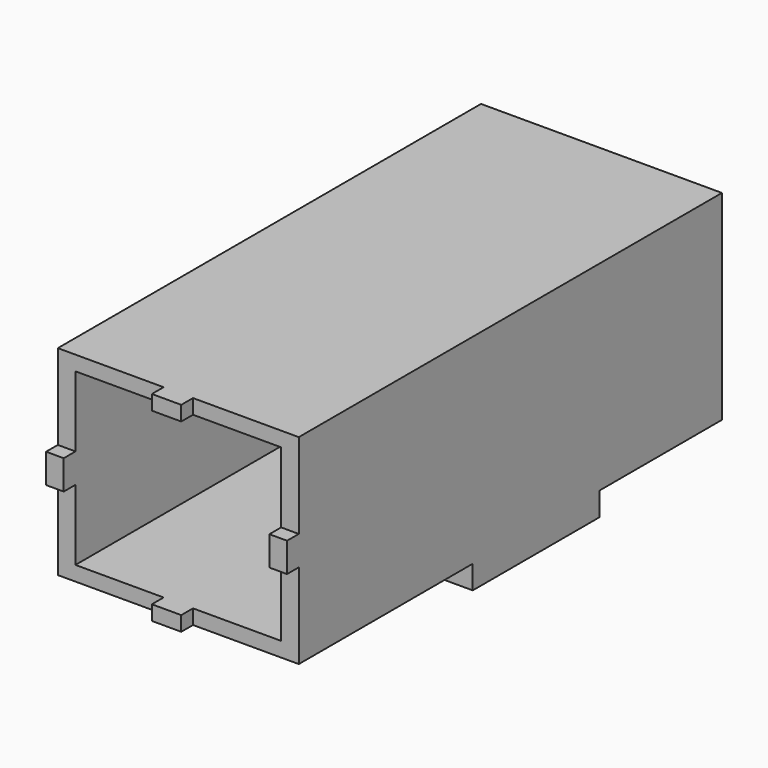
from build123d import *

# Parameters (mm, degrees)
F0_W           = 41
F0_H           = 90
F1_DEPTH       = 34
F2_W           = 35
F2_H           = 29
F3_DEPTH       = 86
F4_W           = 7
F4_H           = 6
F4_R           = 1.55
F4_R_2         = 4
F5_DEPTH       = 4
F6_W           = 5
F6_H           = 2.5
F6_W_2         = 3
F6_H_2         = 5
F7_DEPTH       = 2.5
F8_W           = 5
F8_H           = 27
F9_DEPTH       = 4
F10_T4_DEPTH   = 29
F10_T10_DEPTH  = 29
F10_T16_DEPTH  = 29
F10_T23_DEPTH  = 29
F10_T29_DEPTH  = 29
F10_T35_DEPTH  = 29
F10_T41_DEPTH  = 29
F10_T47_DEPTH  = 29
F10_T54_DEPTH  = 29
F10_T60_DEPTH  = 29
F10_T66_DEPTH  = 35
F10_T72_DEPTH  = 35
F10_T78_DEPTH  = 35
F10_T85_DEPTH  = 35
F10_T91_DEPTH  = 35
F10_T97_DEPTH  = 35
F10_T103_DEPTH = 35
F10_T109_DEPTH = 35
F10_T116_DEPTH = 35
F10_T122_DEPTH = 35


# Not quite as in the source:
# - a fillet or chamfer that OpenCascade refuses, or shapes differently, is made with other operations: its cross-section is extruded or revolved along the edge and cut away or added


with BuildPart() as f1:
    # F0 (on Top) → F1 (new body)
    with BuildSketch(Plane.XY):
        with Locations((-1.7023412511, 4.193077401)):
            Rectangle(F0_W, F0_H)
    extrude(amount=F1_DEPTH)

    # F2 (on face) → F3 (cut)
    with BuildSketch(Plane.XZ.offset(40.806922599)):
        with Locations((-1.7023412511, 17)):
            Rectangle(F2_W, F2_H)
    extrude(amount=-F3_DEPTH, mode=Mode.SUBTRACT)

    # F4 (on face) → F5 (cut, through all)
    with BuildSketch(Plane(origin=(0, 49.193077401, 0), x_dir=(-1, 0, 0), z_dir=(0, 1, 0))):
        with Locations((-11.2976587489, 7)):
            Rectangle(F4_W, F4_H)
        with Locations((-7.7976587489, 17)):
            Circle(F4_R)
        with Locations((1.7023412511, 25)):
            Circle(F4_R)
        with Locations((1.7023412511, 17)):
            Circle(F4_R_2)
        with Locations((1.7023412511, 9)):
            Circle(F4_R)
        with Locations((11.2023412511, 17)):
            Circle(F4_R)
        with Locations((14.7023412511, 27)):
            Rectangle(F4_W, F4_H)
    extrude(amount=-F5_DEPTH, mode=Mode.SUBTRACT)

    # F6 (on face) → F7 (join)
    with BuildSketch(Plane.XZ.offset(40.806922599)):
        with Locations((-1.7023412511, 32.75)):
            Rectangle(F6_W, F6_H)
        with Locations((-20.7023412511, 17)):
            Rectangle(F6_W_2, F6_H_2)
        with Locations((17.2976587489, 17)):
            Rectangle(F6_W_2, F6_H_2)
        with Locations((-1.7023412511, 1.25)):
            Rectangle(F6_W, F6_H)
    extrude(amount=F7_DEPTH)

    # F8 (on face) → F9 (join)
    with BuildSketch(Plane(origin=(0, 0, 0), x_dir=(1, 0, 0), z_dir=(0, 0, -1))):
        with Locations((-19.7023412511, -9.693077401)):
            Rectangle(F8_W, F8_H)
        with Locations((16.2976587489, -9.693077401)):
            Rectangle(F8_W, F8_H)
    extrude(amount=F9_DEPTH)

    # F10: chamfer of 3 on 4 edges, made by hand


with BuildPart() as f10_tool2:
    # F10_s3 → F10_t4 (new body)
    with BuildSketch(Plane.XY.offset(31.5)):
        Polygon((-16.2023412511, 45.193077401), (-19.2023412511, 42.193077401), (-19.2023412511, 45.193077401), align=None)
    extrude(amount=-F10_T4_DEPTH)

    split(bisect_by=Plane.YZ.offset(-18.2023412511), keep=Keep.TOP)

    split(bisect_by=Plane.XY.offset(30), keep=Keep.TOP)


with BuildPart() as f1_1:
    add(f1.part)

    # F10_t1: union F10_tool2
    add(f10_tool2.part)


with BuildPart() as f10_tool8:
    # F10_s9 → F10_t10 (new body)
    with BuildSketch(Plane.XY.offset(31.5)):
        Polygon((-16.2023412511, 45.193077401), (-19.2023412511, 42.193077401), (-19.2023412511, 45.193077401), align=None)
    extrude(amount=-F10_T10_DEPTH)

    split(bisect_by=Plane.YZ.offset(-18.2023412511), keep=Keep.BOTTOM)

    split(bisect_by=Plane.XY.offset(30), keep=Keep.TOP)


with BuildPart() as f1_2:
    add(f1_1.part)

    # F10_t7: union F10_tool8
    add(f10_tool8.part)


with BuildPart() as f10_tool14:
    # F10_s15 → F10_t16 (new body)
    with BuildSketch(Plane.XY.offset(31.5)):
        Polygon((-16.2023412511, 45.193077401), (-19.2023412511, 42.193077401), (-19.2023412511, 45.193077401), align=None)
    extrude(amount=-F10_T16_DEPTH)

    split(bisect_by=Plane.YZ.offset(-18.2023412511), keep=Keep.BOTTOM)

    split(bisect_by=Plane.XY.offset(24), keep=Keep.TOP)

    split(bisect_by=Plane.XY.offset(30), keep=Keep.BOTTOM)


with BuildPart() as f1_3:
    add(f1_2.part)

    # F10_t13: union F10_tool14
    add(f10_tool14.part)


with BuildPart() as f10_tool21:
    # F10_s22 → F10_t23 (new body)
    with BuildSketch(Plane.XY.offset(31.5)):
        Polygon((-16.2023412511, 45.193077401), (-19.2023412511, 42.193077401), (-19.2023412511, 45.193077401), align=None)
    extrude(amount=-F10_T23_DEPTH)

    split(bisect_by=Plane.YZ.offset(-18.2023412511), keep=Keep.TOP)

    split(bisect_by=Plane.XY.offset(24), keep=Keep.BOTTOM)


with BuildPart() as f1_4:
    add(f1_3.part)

    # F10_t20: union F10_tool21
    add(f10_tool21.part)


with BuildPart() as f10_tool27:
    # F10_s28 → F10_t29 (new body)
    with BuildSketch(Plane.XY.offset(31.5)):
        Polygon((-16.2023412511, 45.193077401), (-19.2023412511, 42.193077401), (-19.2023412511, 45.193077401), align=None)
    extrude(amount=-F10_T29_DEPTH)

    split(bisect_by=Plane.YZ.offset(-18.2023412511), keep=Keep.BOTTOM)

    split(bisect_by=Plane.XY.offset(24), keep=Keep.BOTTOM)


with BuildPart() as f1_5:
    add(f1_4.part)

    # F10_t26: union F10_tool27
    add(f10_tool27.part)


with BuildPart() as f10_tool33:
    # F10_s34 → F10_t35 (new body)
    with BuildSketch(Plane.XY.offset(2.5)):
        Polygon((12.7976587489, 45.193077401), (15.7976587489, 42.193077401), (15.7976587489, 45.193077401), align=None)
    extrude(amount=F10_T35_DEPTH)

    split(bisect_by=Plane.XY.offset(4), keep=Keep.BOTTOM)

    split(bisect_by=Plane.YZ.offset(14.7976587489), keep=Keep.BOTTOM)


with BuildPart() as f1_6:
    add(f1_5.part)

    # F10_t32: union F10_tool33
    add(f10_tool33.part)


with BuildPart() as f10_tool39:
    # F10_s40 → F10_t41 (new body)
    with BuildSketch(Plane.XY.offset(2.5)):
        Polygon((12.7976587489, 45.193077401), (15.7976587489, 42.193077401), (15.7976587489, 45.193077401), align=None)
    extrude(amount=F10_T41_DEPTH)

    split(bisect_by=Plane.XY.offset(4), keep=Keep.BOTTOM)

    split(bisect_by=Plane.YZ.offset(14.7976587489), keep=Keep.TOP)


with BuildPart() as f1_7:
    add(f1_6.part)

    # F10_t38: union F10_tool39
    add(f10_tool39.part)


with BuildPart() as f10_tool45:
    # F10_s46 → F10_t47 (new body)
    with BuildSketch(Plane.XY.offset(2.5)):
        Polygon((12.7976587489, 45.193077401), (15.7976587489, 42.193077401), (15.7976587489, 45.193077401), align=None)
    extrude(amount=F10_T47_DEPTH)

    split(bisect_by=Plane.XY.offset(4), keep=Keep.TOP)

    split(bisect_by=Plane.YZ.offset(14.7976587489), keep=Keep.TOP)

    split(bisect_by=Plane.XY.offset(10), keep=Keep.BOTTOM)


with BuildPart() as f1_8:
    add(f1_7.part)

    # F10_t44: union F10_tool45
    add(f10_tool45.part)


with BuildPart() as f10_tool52:
    # F10_s53 → F10_t54 (new body)
    with BuildSketch(Plane.XY.offset(2.5)):
        Polygon((12.7976587489, 45.193077401), (15.7976587489, 42.193077401), (15.7976587489, 45.193077401), align=None)
    extrude(amount=F10_T54_DEPTH)

    split(bisect_by=Plane.YZ.offset(14.7976587489), keep=Keep.BOTTOM)

    split(bisect_by=Plane.XY.offset(10), keep=Keep.TOP)


with BuildPart() as f1_9:
    add(f1_8.part)

    # F10_t51: union F10_tool52
    add(f10_tool52.part)


with BuildPart() as f10_tool58:
    # F10_s59 → F10_t60 (new body)
    with BuildSketch(Plane.XY.offset(2.5)):
        Polygon((12.7976587489, 45.193077401), (15.7976587489, 42.193077401), (15.7976587489, 45.193077401), align=None)
    extrude(amount=F10_T60_DEPTH)

    split(bisect_by=Plane.YZ.offset(14.7976587489), keep=Keep.TOP)

    split(bisect_by=Plane.XY.offset(10), keep=Keep.TOP)


with BuildPart() as f1_10:
    add(f1_9.part)

    # F10_t57: union F10_tool58
    add(f10_tool58.part)


with BuildPart() as f10_tool64:
    # F10_s65 → F10_t66 (new body)
    with BuildSketch(Plane.YZ.offset(15.7976587489)):
        Polygon((45.193077401, 28.5), (42.193077401, 31.5), (45.193077401, 31.5), align=None)
    extrude(amount=-F10_T66_DEPTH)

    split(bisect_by=Plane.YZ.offset(-11.2023412511), keep=Keep.TOP)

    split(bisect_by=Plane.XY.offset(30), keep=Keep.BOTTOM)


with BuildPart() as f1_11:
    add(f1_10.part)

    # F10_t63: union F10_tool64
    add(f10_tool64.part)


with BuildPart() as f10_tool70:
    # F10_s71 → F10_t72 (new body)
    with BuildSketch(Plane.YZ.offset(15.7976587489)):
        Polygon((45.193077401, 28.5), (42.193077401, 31.5), (45.193077401, 31.5), align=None)
    extrude(amount=-F10_T72_DEPTH)

    split(bisect_by=Plane.YZ.offset(-11.2023412511), keep=Keep.TOP)

    split(bisect_by=Plane.XY.offset(30), keep=Keep.TOP)


with BuildPart() as f1_12:
    add(f1_11.part)

    # F10_t69: union F10_tool70
    add(f10_tool70.part)


with BuildPart() as f10_tool76:
    # F10_s77 → F10_t78 (new body)
    with BuildSketch(Plane.YZ.offset(15.7976587489)):
        Polygon((45.193077401, 28.5), (42.193077401, 31.5), (45.193077401, 31.5), align=None)
    extrude(amount=-F10_T78_DEPTH)

    split(bisect_by=Plane.YZ.offset(-18.2023412511), keep=Keep.TOP)

    split(bisect_by=Plane.YZ.offset(-11.2023412511), keep=Keep.BOTTOM)

    split(bisect_by=Plane.XY.offset(30), keep=Keep.TOP)


with BuildPart() as f1_13:
    add(f1_12.part)

    # F10_t75: union F10_tool76
    add(f10_tool76.part)


with BuildPart() as f10_tool83:
    # F10_s84 → F10_t85 (new body)
    with BuildSketch(Plane.YZ.offset(15.7976587489)):
        Polygon((45.193077401, 28.5), (42.193077401, 31.5), (45.193077401, 31.5), align=None)
    extrude(amount=-F10_T85_DEPTH)

    split(bisect_by=Plane.YZ.offset(-18.2023412511), keep=Keep.BOTTOM)

    split(bisect_by=Plane.XY.offset(30), keep=Keep.BOTTOM)


with BuildPart() as f1_14:
    add(f1_13.part)

    # F10_t82: union F10_tool83
    add(f10_tool83.part)


with BuildPart() as f10_tool89:
    # F10_s90 → F10_t91 (new body)
    with BuildSketch(Plane.YZ.offset(15.7976587489)):
        Polygon((45.193077401, 28.5), (42.193077401, 31.5), (45.193077401, 31.5), align=None)
    extrude(amount=-F10_T91_DEPTH)

    split(bisect_by=Plane.YZ.offset(-18.2023412511), keep=Keep.BOTTOM)

    split(bisect_by=Plane.XY.offset(30), keep=Keep.TOP)


with BuildPart() as f1_15:
    add(f1_14.part)

    # F10_t88: union F10_tool89
    add(f10_tool89.part)


with BuildPart() as f10_tool95:
    # F10_s96 → F10_t97 (new body)
    with BuildSketch(Plane.YZ.offset(-19.2023412511)):
        Polygon((45.193077401, 5.5), (42.193077401, 2.5), (45.193077401, 2.5), align=None)
    extrude(amount=F10_T97_DEPTH)

    split(bisect_by=Plane.YZ.offset(7.7976587489), keep=Keep.BOTTOM)

    split(bisect_by=Plane.XY.offset(4), keep=Keep.TOP)


with BuildPart() as f1_16:
    add(f1_15.part)

    # F10_t94: union F10_tool95
    add(f10_tool95.part)


with BuildPart() as f10_tool101:
    # F10_s102 → F10_t103 (new body)
    with BuildSketch(Plane.YZ.offset(-19.2023412511)):
        Polygon((45.193077401, 5.5), (42.193077401, 2.5), (45.193077401, 2.5), align=None)
    extrude(amount=F10_T103_DEPTH)

    split(bisect_by=Plane.YZ.offset(7.7976587489), keep=Keep.BOTTOM)

    split(bisect_by=Plane.XY.offset(4), keep=Keep.BOTTOM)


with BuildPart() as f1_17:
    add(f1_16.part)

    # F10_t100: union F10_tool101
    add(f10_tool101.part)


with BuildPart() as f10_tool107:
    # F10_s108 → F10_t109 (new body)
    with BuildSketch(Plane.YZ.offset(-19.2023412511)):
        Polygon((45.193077401, 5.5), (42.193077401, 2.5), (45.193077401, 2.5), align=None)
    extrude(amount=F10_T109_DEPTH)

    split(bisect_by=Plane.YZ.offset(7.7976587489), keep=Keep.TOP)

    split(bisect_by=Plane.XY.offset(4), keep=Keep.BOTTOM)

    split(bisect_by=Plane.YZ.offset(14.7976587489), keep=Keep.BOTTOM)


with BuildPart() as f1_18:
    add(f1_17.part)

    # F10_t106: union F10_tool107
    add(f10_tool107.part)


with BuildPart() as f10_tool114:
    # F10_s115 → F10_t116 (new body)
    with BuildSketch(Plane.YZ.offset(-19.2023412511)):
        Polygon((45.193077401, 5.5), (42.193077401, 2.5), (45.193077401, 2.5), align=None)
    extrude(amount=F10_T116_DEPTH)

    split(bisect_by=Plane.XY.offset(4), keep=Keep.TOP)

    split(bisect_by=Plane.YZ.offset(14.7976587489), keep=Keep.TOP)


with BuildPart() as f1_19:
    add(f1_18.part)

    # F10_t113: union F10_tool114
    add(f10_tool114.part)


with BuildPart() as f10_tool120:
    # F10_s121 → F10_t122 (new body)
    with BuildSketch(Plane.YZ.offset(-19.2023412511)):
        Polygon((45.193077401, 5.5), (42.193077401, 2.5), (45.193077401, 2.5), align=None)
    extrude(amount=F10_T122_DEPTH)

    split(bisect_by=Plane.XY.offset(4), keep=Keep.BOTTOM)

    split(bisect_by=Plane.YZ.offset(14.7976587489), keep=Keep.TOP)


with BuildPart() as f1_20:
    add(f1_19.part)

    # F10_t119: union F10_tool120
    add(f10_tool120.part)


solid = f1_20.part
